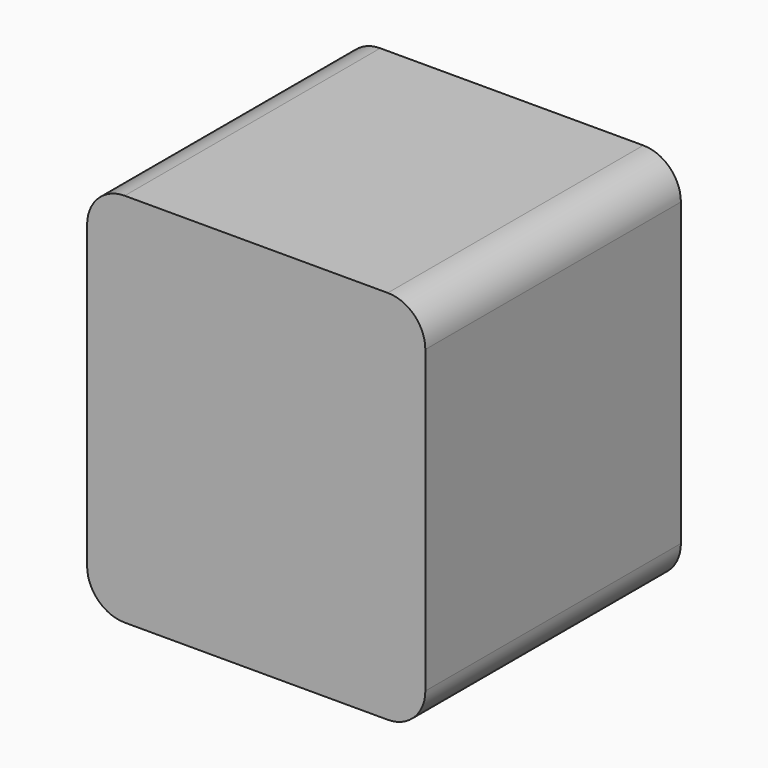
from build123d import *

# Parameters (mm, degrees)
F0_W         = 18
F0_H         = 17
F1_DEPTH     = 20
F2_TEXT_SIZE = 13.6162471285
F3_DEPTH     = 1
F4_TEXT_SIZE = 13.4210716674
F5_DEPTH     = 1
F6_R         = 2


# Not quite as in the source:
# - Text() gives the source's letters only with a copy of the font that has no kerning and outlines rounded to 1/6400 em; it was checked with that copy


with BuildPart() as f1:
    # F0 (on Top) → F1 (new body)
    with BuildSketch(Plane.XY):
        with Locations((-9, 8.5)):
            Rectangle(F0_W, F0_H)
    extrude(amount=F1_DEPTH)

    # F2 (on face) → F3 (cut)
    with BuildSketch(Plane(origin=(0, 17, 0), x_dir=(-1, 0, 0), z_dir=(0, 1, 0))):
        with Locations((1.6068861587, 4.7744796611)):
            Text('18', F2_TEXT_SIZE, font='Open Sans', text_align=(TextAlign.LEFT, TextAlign.BOTTOM))
    extrude(amount=-F3_DEPTH, mode=Mode.SUBTRACT)

    # F4 (on face) → F5 (cut)
    with BuildSketch(Plane(origin=(-18, 0, 0), x_dir=(0, -1, 0), z_dir=(-1, 0, 0))):
        with Locations((-16.3586996496, 5.3555383347)):
            Text('17', F4_TEXT_SIZE, font='Open Sans', text_align=(TextAlign.LEFT, TextAlign.BOTTOM))
    extrude(amount=-F5_DEPTH, mode=Mode.SUBTRACT)

    # F6
    f6_edges = [f1.edges().sort_by_distance(p)[0] for p in [
        (0, 8.5, 0),
        (0, 8.5, 20),
        (-18, 8.5, 0),
        (-18, 8.5, 20),
    ]]
    fillet(f6_edges, radius=F6_R)


solid = f1.part
